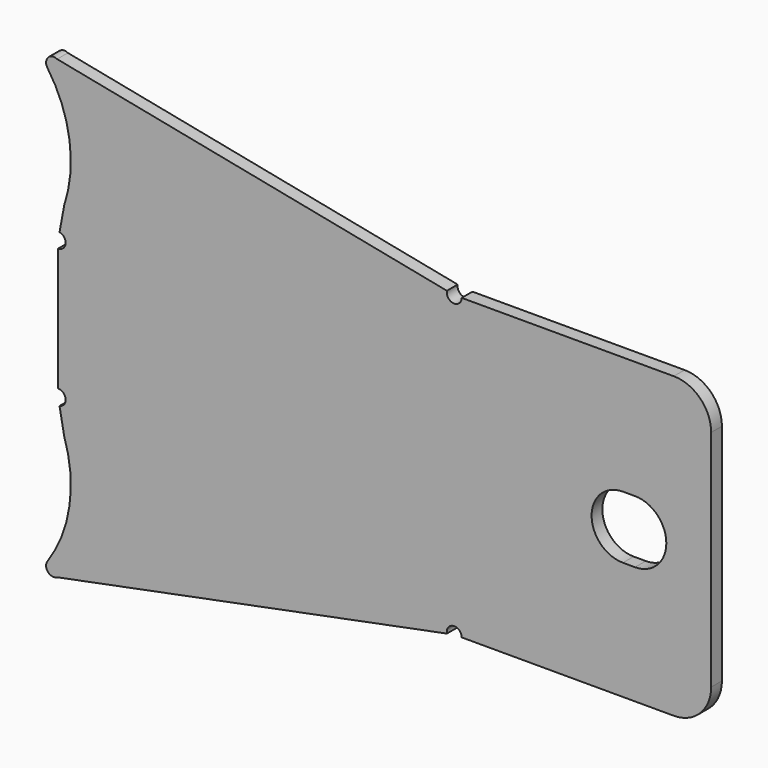
from build123d import *

# Parameters (mm, degrees)
F1_DEPTH = 2.286


# Not quite as in the source:
# - ends of sketch curves that miss each other by under 0.0002 mm in the source are joined


with BuildPart() as f1:
    # F0 (on Front) → F1 (new body)
    with BuildSketch(Plane.XZ):
        with BuildLine():
            ThreePointArc((-20.1784623574, -17.2534296725), (-19.281646508, -27.4231568168), (-23.0260908036, -36.9208810585))
            ThreePointArc((-23.0260908036, -36.9208810585), (-22.9304929279, -38.4914502694), (-21.3807341969, -38.7636168977))
            Line((-21.3807341969, -38.7636168977), (44.86735167, -25.6466681175))
            ThreePointArc((44.86735167, -25.6466681175), (45.9892411408, -24.1360607291), (47.3831666, -25.4))
            Line((47.3831666, -25.4), (76.8344666, -5.3213))
            Line((76.8344666, -5.3213), (74.7770666, -5.3213))
            ThreePointArc((74.7770666, -5.3213), (69.4557666, 0), (74.7770666, 5.3213))
            Line((74.7770666, 5.3213), (76.8344666, 5.3213))
            Line((76.8344666, 5.3213), (47.3831666, 25.4))
            ThreePointArc((47.3831666, 25.4), (45.9892409445, 24.1360607483), (44.8673517466, 25.6466685044))
            Line((44.8673517466, 25.6466685044), (-21.38072359, 38.7636365822))
            ThreePointArc((-21.38072359, 38.7636365822), (-22.9304889155, 38.4914801631), (-23.026090887, 36.9209064006))
            ThreePointArc((-23.026090887, 36.9209064006), (-19.281646508, 27.4231822168), (-20.1784623574, 17.2534550725))
            Line((-20.1784623574, 17.2534550725), (-20.9658562769, 12.9963192698))
            ThreePointArc((-20.9658562769, 12.9963192698), (-19.9321396678, 11.6315268838), (-21.1968334, 10.4775))
            Line((-21.1968334, 10.4775), (-21.1968334, -10.4775))
            ThreePointArc((-21.1968334, -10.4775), (-19.9321397156, -11.6315263621), (-20.9658552466, -12.9963190792))
            Line((-20.9658552466, -12.9963190792), (-20.1784623574, -17.2534296725))
        make_face()
        with BuildLine():
            Line((76.8344666, -5.3213), (47.3831666, -25.4))
            Line((47.3831666, -25.4), (83.4257666, -25.4))
            ThreePointArc((83.4257666, -25.4), (87.9158946605, -23.5401280605), (89.7757666, -19.05))
            Line((89.7757666, -19.05), (89.7757666, 19.05))
            ThreePointArc((89.7757666, 19.05), (87.9158946605, 23.5401280605), (83.4257666, 25.4))
            Line((83.4257666, 25.4), (47.3831666, 25.4))
            Line((47.3831666, 25.4), (76.8344666, 5.3213))
            ThreePointArc((76.8344666, 5.3213), (82.1557666, 0), (76.8344666, -5.3213))
        make_face()
    extrude(amount=F1_DEPTH)


solid = f1.part
